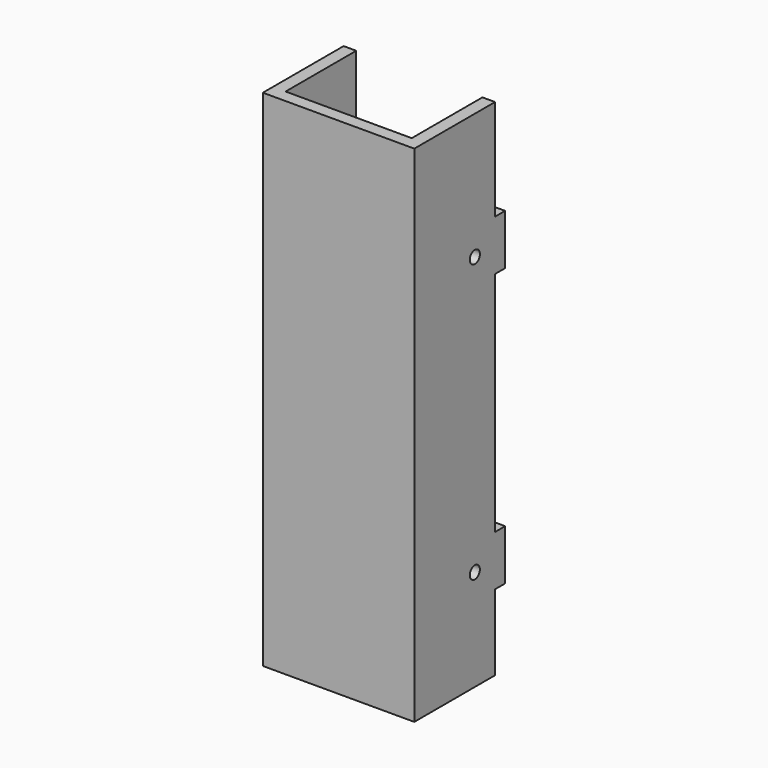
from build123d import *

# Parameters (mm, degrees)
F2_DEPTH = 200
F3_W     = 5
F3_H     = 20
F4_DEPTH = 5
F5_W     = 5
F5_H     = 20
F6_DEPTH = 5
F7_D     = 5


with BuildPart() as f2:
    # F1 (on Top) → F2 (new body)
    with BuildSketch(Plane.XY):
        Polygon((30, -55), (30, -15), (25, -15), (25, -50), (-25, -50), (-25, -15), (-30, -15), (-30, -55), align=None)
    extrude(amount=F2_DEPTH)

    # F3 (on face) → F4 (join)
    with BuildSketch(Plane.YZ.offset(30)):
        with Locations((-12.5, 150)):
            Rectangle(F3_W, F3_H)
        with Locations((-12.5, 40)):
            Rectangle(F3_W, F3_H)
    extrude(amount=-F4_DEPTH)

    # F5 (on face) → F6 (join)
    with BuildSketch(Plane(origin=(-30, 0, 0), x_dir=(0, -1, 0), z_dir=(-1, 0, 0))):
        with Locations((12.5, 150)):
            Rectangle(F5_W, F5_H)
        with Locations((12.5, 40)):
            Rectangle(F5_W, F5_H)
    extrude(amount=-F6_DEPTH)

    # F7 (through all)
    with Locations(Plane.YZ.offset(30)):
        with Locations((-25, 150), (-25, 40)):
            Hole(F7_D / 2)


solid = f2.part
